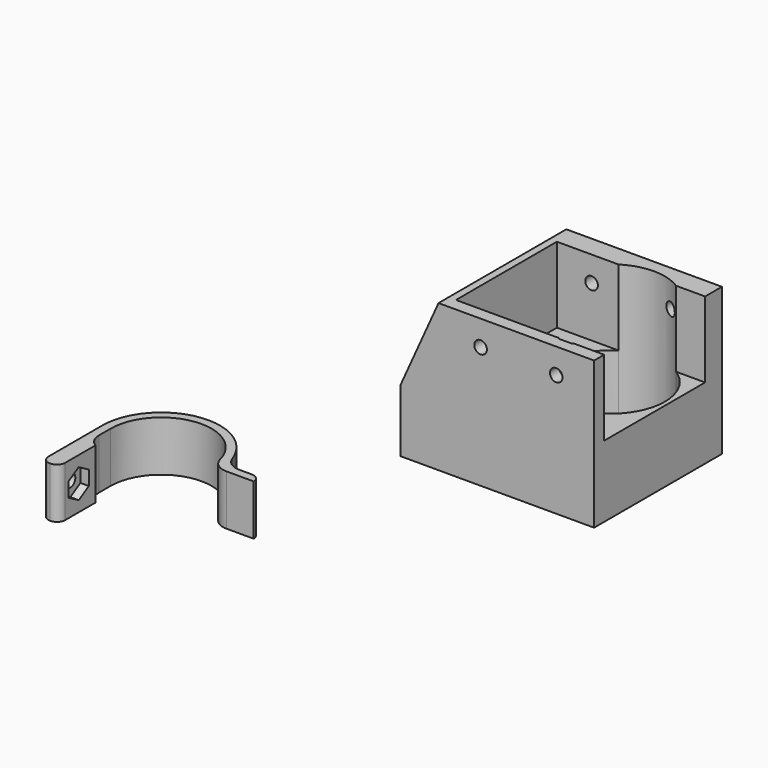
from build123d import *

# Parameters (mm, degrees)
F0_W         = 46
F0_H         = 36
F1_DEPTH     = 35
F2_R         = 1.5
F3_DEPTH     = 50
F4_DEPTH     = 30
F6_DEPTH     = 18
F8_DEPTH     = 25
F9_R         = 1.5
F10_DEPTH    = 50
F11_T1_DEPTH = 139.6606830198
F13_DEPTH    = 6
F14_W        = 11
F14_H        = 12
F15_DEPTH    = 2
F14_R        = 1.5
F16_DEPTH    = 25
F17_T1_DEPTH = 12
F17_T3_DEPTH = 12
F17_T5_DEPTH = 29.4596669241
F18_R        = 1.99999
F19_DEPTH    = 2


# Not quite as in the source:
# - a fillet or chamfer that OpenCascade refuses, or shapes differently, is made with other operations: its cross-section is extruded or revolved along the edge and cut away or added
# - a fillet or chamfer is up to 0.001 mm smaller than in the source, because OpenCascade refuses the exact size
# - a feature names something its author has since deleted; it is built from what else it names


with BuildPart() as f1:
    # F0 (on Top) → F1 (new body)
    with BuildSketch(Plane.XY):
        Rectangle(F0_W, F0_H)
    extrude(amount=F1_DEPTH)

    # F2 (on face) → F3 (cut)
    with BuildSketch(Plane.XY.offset(35)):
        with Locations((-18, 13)):
            Circle(F2_R)
        with Locations((-18, -13)):
            Circle(F2_R)
        with Locations((14, -12.5)):
            Circle(F2_R)
    extrude(amount=-F3_DEPTH, mode=Mode.SUBTRACT)

    # F2 (on face) → F4 (cut)
    with BuildSketch(Plane.XY.offset(35)):
        Polygon((10.8247584463, -12.5342696548), (12.4420576148, -15.266974676), (15.6172991685, -15.2327050212), (17.1752415537, -12.4657303452), (15.5579423852, -9.733025324), (12.3827008315, -9.7672949788), align=None)
        with Locations((14, -12.5)):
            Circle(F2_R, mode=Mode.SUBTRACT)
        Polygon((-14.8246241, -13.01792281), (-16.3967904413, -10.259005209), (-19.5721663413, -10.2410823991), (-21.1753759, -12.98207719), (-19.6032095587, -15.740994791), (-16.4278336587, -15.7589176009), align=None)
        with Locations((-18, -13)):
            Circle(F2_R, mode=Mode.SUBTRACT)
        Polygon((-19.5877132403, 15.75), (-21.1754264805, 13), (-19.5877132403, 10.25), (-16.4122867597, 10.25), (-14.8245735195, 13), (-16.4122867597, 15.75), align=None)
        with Locations((-18, 13)):
            Circle(F2_R, mode=Mode.SUBTRACT)
    extrude(amount=-F4_DEPTH, mode=Mode.SUBTRACT)

    # F5 (on face) → F6 (cut)
    with BuildSketch(Plane.XY.offset(35)):
        Polygon((15.7483235031, -15), (23, -15), (23, 15), (-12.25, 15), (-12.25, -15), (12.2840537621, -15), (10.8247584463, -12.5342696548), (12.3827008315, -9.7672949788), (15.5579423852, -9.733025324), (17.1752415537, -12.4657303452), align=None)
    extrude(amount=-F6_DEPTH, mode=Mode.SUBTRACT)

    # F7 (on face) → F8 (cut, symmetric)
    with BuildSketch(Plane.XY.offset(17)):
        with BuildLine():
            Line((2.3943453996, 15), (16.1056546004, 15))
            ThreePointArc((16.1056546004, 15), (9.25, 17), (2.3943453996, 15))
        make_face()
        with BuildLine():
            ThreePointArc((2.3943453996, 15), (3.120036548, -6.9297159211), (22, 4.25))
            ThreePointArc((22, 4.25), (20.4297159211, 10.379963452), (16.1056546004, 15))
            Line((16.1056546004, 15), (2.3943453996, 15))
        make_face()
    extrude(amount=F8_DEPTH, both=True, mode=Mode.SUBTRACT)

    # F9 (on face) → F10 (cut, symmetric)
    with BuildSketch(Plane.XZ.offset(-15)):
        with Locations((14, 29)):
            Circle(F9_R)
        with Locations((-4, 29)):
            Circle(F9_R)
    extrude(amount=F10_DEPTH, both=True, mode=Mode.SUBTRACT)

    # F11: chamfer of 9 x 20 on 1 edges, made by hand

    # F11_s2 → F11_t1 (cut)
    with BuildSketch(Plane.XZ.offset(-69.8303415099)):
        Polygon((-14, 35), (-23, 15), (-23, 35), align=None)
    extrude(amount=F11_T1_DEPTH, mode=Mode.SUBTRACT)

    # F19 (add): a face of the model
    f19_faces = [f1.faces().sort_by_distance(p)[0] for p in [
        (1.1483875738, 18, 16.7445677024),
    ]]
    extrude(f19_faces, amount=F19_DEPTH)


with BuildPart() as f13:
    # F12 (on Top) → F13 (new body, symmetric)
    with BuildSketch(Plane.XY):
        with BuildLine():
            ThreePointArc((-64.8061240633, -51.9561834335), (-52.8061240633, -39.9561834335), (-40.8061240633, -51.9561834335))
            Line((-40.8061240633, -51.9561834335), (-40.8061240633, -49.9561834335))
            Line((-40.8061240633, -49.9561834335), (-38.9497176027, -49.9561834335))
            ThreePointArc((-38.9497176027, -49.9561834335), (-53.8086981384, -37.9921279616), (-66.8061240633, -51.9561834335))
            Line((-66.8061240633, -51.9561834335), (-64.8061240633, -51.9561834335))
        make_face()
        with BuildLine():
            ThreePointArc((-38.9497176027, -49.9561834335), (-38.8420685913, -50.9536093584), (-38.8061240633, -51.9561834335))
            Line((-38.8061240633, -51.9561834335), (-30.8061240633, -51.9561834335))
            Line((-30.8061240633, -51.9561834335), (-30.8061240633, -49.9561834335))
            Line((-30.8061240633, -49.9561834335), (-38.9497176027, -49.9561834335))
        make_face()
        with BuildLine():
            Line((-40.8061240633, -49.9561834335), (-40.8061240633, -51.9561834335))
            Line((-40.8061240633, -51.9561834335), (-38.8061240633, -51.9561834335))
            ThreePointArc((-38.8061240633, -51.9561834335), (-38.8420685913, -50.9536093584), (-38.9497176027, -49.9561834335))
            Line((-38.9497176027, -49.9561834335), (-40.8061240633, -49.9561834335))
        make_face()
        with BuildLine():
            Line((-64.8061240633, -59.1672859845), (-64.8061240633, -51.9561834335))
            Line((-64.8061240633, -51.9561834335), (-66.8061240633, -51.9561834335))
            ThreePointArc((-66.8061240633, -51.9561834335), (-66.2968616265, -55.6978408203), (-64.8061240633, -59.1672859845))
        make_face()
        with BuildLine():
            ThreePointArc((-64.8061240633, -59.1672859845), (-66.2968616265, -55.6978408203), (-66.8061240633, -51.9561834335))
            Line((-66.8061240633, -51.9561834335), (-66.8061240633, -69.9561834335))
            Line((-66.8061240633, -69.9561834335), (-64.8061240633, -69.9561834335))
            Line((-64.8061240633, -69.9561834335), (-64.8061240633, -59.1672859845))
        make_face()
    extrude(amount=F13_DEPTH, both=True)

    # F14 (on face) → F15 (join)
    with BuildSketch(Plane.YZ.offset(-64.8061240633)):
        with Locations((-64.4561834335, 0)):
            Rectangle(F14_W, F14_H)
        Polygon((-60.9620828312, 1.742268864), (-60.9502840359, -1.7218327511), (-63.9443846382, -3.4641016151), (-66.9502840359, -1.742268864), (-66.9620828312, 1.7218327511), (-63.9679822288, 3.4641016151), align=None, mode=Mode.SUBTRACT)
    extrude(amount=F15_DEPTH)

    # F14 (on face) → F16 (cut)
    with BuildSketch(Plane.YZ.offset(-64.8061240633)):
        with Locations((-63.9561834335, 0)):
            Circle(F14_R)
    extrude(amount=-F16_DEPTH, mode=Mode.SUBTRACT)

    # F17: fillet of radius 4 on 3 edges, made by hand

    # F17_s2 → F17_t1 (join)
    with BuildSketch(Plane.XY.offset(-6)):
        with BuildLine():
            ThreePointArc((-64.8061240633, -55.4920818184), (-64.2702256784, -57.4920818184), (-62.8061240633, -58.9561834335))
            Line((-62.8061240633, -58.9561834335), (-64.8061240633, -58.9561834335))
            Line((-64.8061240633, -58.9561834335), (-64.8061240633, -55.4920818184))
        make_face()
    extrude(amount=F17_T1_DEPTH)

    # F17_s4 → F17_t3 (join)
    with BuildSketch(Plane.XY.offset(-6)):
        with BuildLine():
            ThreePointArc((-35.8355613148, -49.9561834335), (-38.1449623915, -49.2221697572), (-39.6067974811, -47.2895167669))
            ThreePointArc((-39.6067974811, -47.2895167669), (-39.2127083631, -48.6066984578), (-38.9497176027, -49.9561834335))
            Line((-38.9497176027, -49.9561834335), (-35.8355613148, -49.9561834335))
        make_face()
    extrude(amount=F17_T3_DEPTH)

    # F17_s6 → F17_t5 (cut)
    with BuildSketch(Plane.XY.offset(-14.7298334621)):
        with BuildLine():
            ThreePointArc((-41.1871740246, -48.9561834335), (-39.7636804212, -51.1184610937), (-37.3141906784, -51.9561834335))
            Line((-37.3141906784, -51.9561834335), (-40.8061240633, -51.9561834335))
            ThreePointArc((-40.8061240633, -51.9561834335), (-40.9017677081, -50.4441319237), (-41.1871740246, -48.9561834335))
        make_face()
    extrude(amount=F17_T5_DEPTH, mode=Mode.SUBTRACT)

    # F18 (radius 2 in the source; OpenCascade refuses exactly that, so slightly less here)
    f18_edges = [f13.edges().sort_by_distance(p)[0] for p in [
        (-66.806124, -69.956183, 0),
        (-62.806124, -69.956183, 0),
        (-30.806124, -49.956183, 0),
    ]]
    fillet(f18_edges, radius=F18_R)


solid = Compound([f1.part, f13.part])
